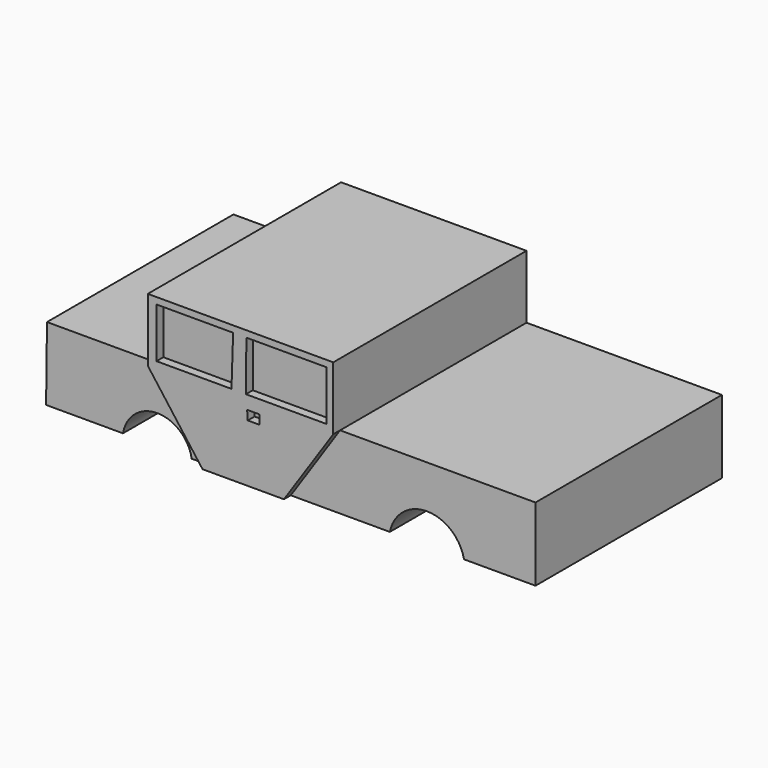
from build123d import *

# Parameters (mm, degrees)
F1_DEPTH = 76.2
F2_W     = 30.3190927953
F2_H     = 20.7057222724
F4_DEPTH = 2.794


# Not quite as in the source:
# - the program builds the solid bodies; features that only make, move or delete a surface that nothing else refers to are left out


with BuildPart() as f1:
    # F0 (on Front) → F1 (new body)
    with BuildSketch(Plane.XZ):
        Polygon((-93.7673449516, 21.5931143612), (-93.7673449516, 21.2973169982), (-93.7673449516, 12.9849165678), (-76.1796534061, -2.6621618308), (-63.4482521564, -2.6621618308), (-63.4482521564, 21.4452156797), align=None)
        Polygon((-63.4482521564, 42.0030392706), (-63.4482521564, 21.4452156797), (-33.1291593611, 21.2973169982), (-33.1291593611, 42.0030392706), align=None)
        Polygon((-93.7673449516, 42.0030392706), (-93.7673449516, 21.5931143612), (-63.4482521564, 21.4452156797), (-63.4482521564, 42.0030392706), align=None)
        with BuildLine():
            Line((30.7627860457, 21.2973169982), (-33.1291593611, 21.2973169982))
            Line((-33.1291593611, 21.2973169982), (-47.1545420587, -2.6621618308))
            Line((-47.1545420587, -2.6621618308), (-16.8603751808, -2.6621618308))
            ThreePointArc((-16.8603751808, -2.6621618308), (-4.7327380162, 7.2386136425), (7.3948991485, -2.6621618308))
            Line((7.3948991485, -2.6621618308), (30.7627860457, -2.6621618308))
            Line((30.7627860457, -2.6621618308), (30.7627860457, 21.2973169982))
        make_face()
        with BuildLine():
            Line((-93.7673449516, 21.2973169982), (-128.96707654, 21.2973169982))
            Line((-128.96707654, 21.2973169982), (-129.2628794909, -2.6621618308))
            Line((-129.2628794909, -2.6621618308), (-104.1202098131, -2.6621618308))
            ThreePointArc((-104.1202098131, -2.6621618308), (-92.8799584508, 6.8226352019), (-81.6397070885, -2.6621618308))
            Line((-81.6397070885, -2.6621618308), (-76.1796534061, -2.6621618308))
            Line((-76.1796534061, -2.6621618308), (-93.7673449516, 12.9849165678))
            Line((-93.7673449516, 12.9849165678), (-93.7673449516, 21.2973169982))
        make_face()
        Polygon((-33.1291593611, 21.2973169982), (-63.4482521564, 21.4452156797), (-63.4482521564, -2.6621618308), (-47.1545420587, -2.6621618308), align=None)
    extrude(amount=F1_DEPTH)

    # F2 (on face) → F4 (join)
    with BuildSketch(Plane.XZ.offset(76.2)):
        with Locations((-78.607798554, 31.6501781344)):
            Rectangle(F2_W, F2_H)
        Polygon((-90.9339487553, 39.8703143001), (-65.8644288778, 39.8703143001), (-66.4106756449, 23.5412772745), (-90.9339487553, 23.5412772745), align=None, mode=Mode.SUBTRACT)
        with Locations((-48.2887057588, 31.6501781344)):
            Rectangle(F2_W, F2_H)
        Polygon((-35.3044308722, 23.5412772745), (-61.6788230836, 23.5412772745), (-61.5411959589, 39.8703143001), (-35.3044308722, 39.8703143001), align=None, mode=Mode.SUBTRACT)
        Polygon((-63.4482521564, 21.2973169982), (-93.7673449516, 21.2973169982), (-75.8718252182, -2.6621618308), (-63.4482521564, -2.6621618308), align=None)
        Polygon((-33.1291593611, 21.2973169982), (-63.4482521564, 21.2973169982), (-63.4482521564, -2.6621618308), (-49.2500411347, -2.6621618308), align=None)
        Polygon((-57.2931170464, 16.1802023649), (-61.0887669027, 16.1802023649), (-61.2885393202, 19.1765353084), (-57.2931170464, 19.1765353084), align=None, mode=Mode.SUBTRACT)
    extrude(amount=F4_DEPTH)


solid = f1.part
